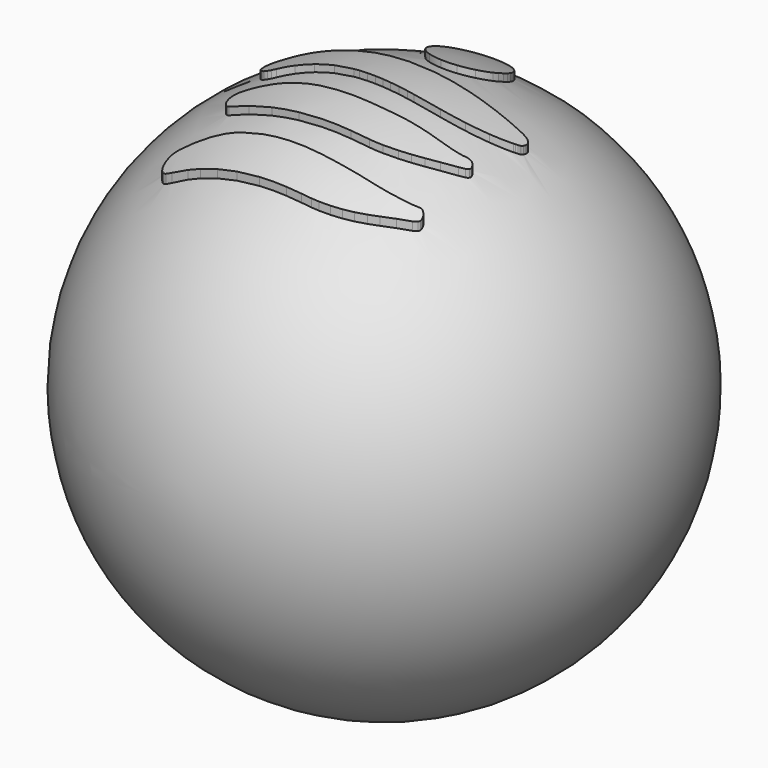
from build123d import *

# Parameters (mm, degrees)
F2_SCALE  = 33.3
F4_DEPTH  = 350
F5_SCALE  = 0.03
F8_SCALE  = 1.4
F9_R      = 2
F10_DEPTH = 25


# Not quite as in the source:
# - ends of sketch curves that miss each other by under 0.0002 mm in the source are joined


with BuildPart() as f1:
    # F0 (on Top) → F1 (revolve)
    with BuildSketch(Plane.XY):
        with BuildLine():
            ThreePointArc((0, 10), (-10, 0), (0, -10))
            Line((0, -10), (0, 10))
        make_face()
    revolve(axis=Axis((0, 0, 0), (0, 1, 0)))


with BuildPart() as f1_1:
    # F2: moved
    add(f1.part.scale(F2_SCALE))

    # F3 (on Top) → F4 (join)
    with BuildSketch(Plane.XY):
        with BuildLine():
            ThreePointArc((12.2771709421, 171.2973365957), (3.7569620218, 171.6476586922), (-4.6595689443, 170.277004793))
            ThreePointArc((-4.6595689443, 170.277004793), (-7.5791100861, 169.3858337465), (-10.4323080104, 168.3008600248))
            ThreePointArc((-10.4323080104, 168.3008600248), (-13.1062595865, 167.0608763501), (-15.6804411014, 165.6252001669))
            ThreePointArc((-15.6804411014, 165.6252001669), (-18.1927436184, 163.9705598843), (-20.5780995786, 162.1376454911))
            ThreePointArc((-20.5780995786, 162.1376454911), (-23.0057078919, 160.0044919193), (-25.3039240862, 157.7325260822))
            ThreePointArc((-25.3039240862, 157.7325260822), (-31.4706435539, 149.5429428278), (-35.5823828621, 140.1519202632))
            ThreePointArc((-35.5823828621, 140.1519202632), (-37.4151892223, 130.0698191221), (-36.8703758239, 119.8369740302))
            ThreePointArc((-36.8703758239, 119.8369740302), (-33.9846977784, 110.064148575), (-28.9042597875, 101.231006158))
            ThreePointArc((-28.9042597875, 101.231006158), (-21.9341856583, 93.8809503165), (-13.4222481029, 88.3898507888))
            ThreePointArc((-13.4222481029, 88.3898507888), (-4.5185212712, 85.102515885), (4.8600680158, 83.6447832896))
            ThreePointArc((4.8600680158, 83.6447832896), (14.0939838139, 84.1373624142), (23.0089839769, 86.5930920584))
            ThreePointArc((23.0089839769, 86.5930920584), (31.1392203878, 90.8795330247), (38.1542056195, 96.8179083614))
            ThreePointArc((38.1542056195, 96.8179083614), (43.8705462201, 104.2320953563), (47.9516467312, 112.6577310976))
            ThreePointArc((47.9516467312, 112.6577310976), (48.8982272616, 115.6703959892), (49.5778582503, 118.7542679562))
            ThreePointArc((49.5778582503, 118.7542679562), (50.0798461554, 122.2623063465), (50.3633334308, 125.7947219788))
            ThreePointArc((50.3633334308, 125.7947219788), (50.4261018055, 129.3073679001), (50.2697793114, 132.8170950236))
            ThreePointArc((50.2697793114, 132.8170950236), (49.8951754848, 135.8589541026), (49.2377071499, 138.8524420404))
            ThreePointArc((49.2377071499, 138.8524420404), (46.1875865729, 146.903977746), (41.6119908777, 154.1974259052))
            ThreePointArc((41.6119908777, 154.1974259052), (35.6444598617, 160.535838967), (28.5782016668, 165.6206104285))
            ThreePointArc((28.5782016668, 165.6206104285), (20.7020851759, 169.246924922), (12.2771709421, 171.2973365957))
        make_face()
        with BuildLine():
            ThreePointArc((-33.4008129923, 51.5219321661), (-43.3379692113, 51.2871840578), (-53.2641999456, 50.7655291885))
            ThreePointArc((-53.2641999456, 50.7655291885), (-64.0634546333, 49.7946073584), (-74.8074670149, 48.3342000935))
            ThreePointArc((-74.8074670149, 48.3342000935), (-84.6019065539, 46.4806697779), (-94.2713978098, 44.0583653252))
            ThreePointArc((-94.2713978098, 44.0583653252), (-102.9502181591, 41.3096782732), (-111.4351770957, 38.0107882245))
            ThreePointArc((-111.4351770957, 38.0107882245), (-118.9134806404, 34.4416572483), (-126.0622642904, 30.2513574505))
            ThreePointArc((-126.0622642904, 30.2513574505), (-129.4839108419, 27.8830120895), (-132.7427949411, 25.2952719306))
            ThreePointArc((-132.7427949411, 25.2952719306), (-136.5624533286, 21.9314871763), (-140.2579578012, 18.4317607976))
            ThreePointArc((-140.2579578012, 18.4317607976), (-143.6296449821, 15.0083482177), (-146.8849228402, 11.4740598577))
            ThreePointArc((-146.8849228402, 11.4740598577), (-148.6323854344, 9.2041815586), (-150.0384499195, 6.708393962))
            ThreePointArc((-150.0384499195, 6.708393962), (-151.1248140292, 3.7850161288), (-151.6963890826, 0.7191350082))
            ThreePointArc((-151.6963890826, 0.7191350082), (-151.7030139521, -2.2793436124), (-151.1351933539, -5.2235748094))
            ThreePointArc((-151.1351933539, -5.2235748094), (-150.0467353665, -7.8799584996), (-148.4426870406, -10.2607450339))
            ThreePointArc((-148.4426870406, -10.2607450339), (-146.4179490275, -12.215036049), (-144.0207902095, -13.6889584416))
            ThreePointArc((-144.0207902095, -13.6889584416), (-142.0108708561, -14.4907449782), (-139.9155901202, -15.0315186278))
            ThreePointArc((-139.9155901202, -15.0315186278), (-137.7958970772, -15.293695428), (-135.6601379416, -15.2745057775))
            ThreePointArc((-135.6601379416, -15.2745057775), (-133.3645757175, -14.9639575717), (-131.1220680921, -14.3832637152))
            ThreePointArc((-131.1220680921, -14.3832637152), (-128.6064090717, -13.4609337915), (-126.1693221699, -12.3474526631))
            ThreePointArc((-126.1693221699, -12.3474526631), (-117.4563433673, -8.4118226468), (-108.438275266, -5.2369791266))
            ThreePointArc((-108.438275266, -5.2369791266), (-98.1841126833, -2.4617275134), (-87.7763850745, -0.3335645669))
            ThreePointArc((-87.7763850745, -0.3335645669), (-76.345030466, 1.2950565214), (-64.8387360221, 2.2612154025))
            ThreePointArc((-64.8387360221, 2.2612154025), (-52.5535288324, 2.6415600166), (-40.2641999843, 2.433295384))
            ThreePointArc((-40.2641999843, 2.433295384), (-36.3905832333, 2.2574401909), (-32.5186950296, 2.0469324971))
            ThreePointArc((-32.5186950296, 2.0469324971), (-27.3626976167, 1.7334768445), (-22.2079499558, 1.4000996639))
            ThreePointArc((-22.2079499558, 1.4000996639), (-16.7235702373, 1.0242285256), (-11.2406670531, 0.6274002856))
            ThreePointArc((-11.2406670531, 0.6274002856), (-6.2514307284, 0.2440051169), (-1.2641999653, -0.1646515892))
            ThreePointArc((-1.2641999653, -0.1646515892), (3.8101984491, -0.5833479876), (8.8862039893, -0.9820881394))
            ThreePointArc((8.8862039893, -0.9820881394), (14.639141156, -1.4147968145), (20.3932289958, -1.8319250593))
            ThreePointArc((20.3932289958, -1.8319250593), (25.9302711121, -2.2181900783), (31.4683470454, -2.5893383091))
            ThreePointArc((31.4683470454, -2.5893383091), (35.8161186925, -2.8625927177), (40.1653459756, -3.111607448))
            ThreePointArc((40.1653459756, -3.111607448), (56.9461627797, -3.5511784434), (73.7250590157, -3.0435602691))
            ThreePointArc((73.7250590157, -3.0435602691), (87.9842368242, -1.5615103417), (102.051928967, 1.1990441357))
            ThreePointArc((102.051928967, 1.1990441357), (114.1685337399, 4.8311708126), (125.8390411692, 9.7100756482))
            ThreePointArc((125.8390411692, 9.7100756482), (136.1926279762, 15.5230963814), (145.7300484377, 22.5959726658))
            ThreePointArc((145.7300484377, 22.5959726658), (146.550290507, 23.3101400968), (147.3486982293, 24.0486367595))
            ThreePointArc((147.3486982293, 24.0486367595), (148.1402478445, 24.8249059327), (148.9094560487, 25.6233189544))
            ThreePointArc((148.9094560487, 25.6233189544), (149.5709024329, 26.3502366545), (150.2112826843, 27.0957792634))
            ThreePointArc((150.2112826843, 27.0957792634), (150.6030770817, 27.6129066708), (150.9446144028, 28.1645187761))
            ThreePointArc((150.9446144028, 28.1645187761), (151.5239999447, 29.4421682368), (151.887939637, 30.7970200663))
            ThreePointArc((151.887939637, 30.7970200663), (152.1005515096, 32.4270102974), (152.1458885281, 34.0701829889))
            ThreePointArc((152.1458885281, 34.0701829889), (152.0249488316, 35.6774007081), (151.7389896858, 37.2635919264))
            ThreePointArc((151.7389896858, 37.2635919264), (151.3206994021, 38.5039844833), (150.6750962556, 39.642728179))
            ThreePointArc((150.6750962556, 39.642728179), (149.4466397487, 41.0713121268), (147.9606871699, 42.2297172692))
            ThreePointArc((147.9606871699, 42.2297172692), (146.1844598756, 43.1548672571), (144.2800719274, 43.7746996926))
            ThreePointArc((144.2800719274, 43.7746996926), (141.3104289541, 44.3482005482), (138.3037060219, 44.6757673241))
            ThreePointArc((138.3037060219, 44.6757673241), (132.5218972582, 45.0258497218), (126.7358000073, 45.2959401848))
            ThreePointArc((126.7358000073, 45.2959401848), (122.2434994951, 45.4817627119), (117.7518210141, 45.6820583056))
            ThreePointArc((117.7518210141, 45.6820583056), (110.7327238683, 46.0095574172), (103.7139249982, 46.3433879632))
            ThreePointArc((103.7139249982, 46.3433879632), (95.7766243193, 46.7281179043), (87.8396770147, 47.1200702955))
            ThreePointArc((87.8396770147, 47.1200702955), (80.0375486713, 47.5126727242), (72.2358000183, 47.9127493529))
            ThreePointArc((72.2358000183, 47.9127493529), (47.9771765909, 49.1252386442), (23.714403985, 50.2516516642))
            ThreePointArc((23.714403985, 50.2516516642), (7.3055536967, 50.8943151333), (-9.1093480016, 51.3573339307))
            ThreePointArc((-9.1093480016, 51.3573339307), (-21.2544240802, 51.5365077254), (-33.4008129923, 51.5219321661))
        make_face()
        with BuildLine():
            ThreePointArc((135.3719059726, -35.3477778582), (133.7818150804, -35.7341828726), (132.2357999771, -36.2704059429))
            ThreePointArc((132.2357999771, -36.2704059429), (128.8416633612, -37.4833877287), (125.3645320803, -38.4326223458))
            ThreePointArc((125.3645320803, -38.4326223458), (121.5804634451, -39.1872771875), (117.7566089761, -39.7038197692))
            ThreePointArc((117.7566089761, -39.7038197692), (112.4926277716, -40.144911978), (107.2155060146, -40.3816535735))
            ThreePointArc((107.2155060146, -40.3816535735), (98.4763113976, -40.5631318855), (89.7358000012, -40.6627181729))
            ThreePointArc((89.7358000012, -40.6627181729), (84.01711687, -40.7186101274), (78.2988839889, -40.8095684171))
            ThreePointArc((78.2988839889, -40.8095684171), (72.2794587222, -40.9395955211), (66.2608000019, -41.101258064))
            ThreePointArc((66.2608000019, -41.101258064), (60.7936656268, -41.2769639411), (55.3275380245, -41.4816096107))
            ThreePointArc((55.3275380245, -41.4816096107), (51.5300788633, -41.6626782072), (47.7357999863, -41.9012778052))
            ThreePointArc((47.7357999863, -41.9012778052), (43.1515752062, -42.1702788658), (38.5622899772, -42.3313360205))
            ThreePointArc((38.5622899772, -42.3313360205), (33.1237885443, -42.4194447684), (27.6845839986, -42.4301682736))
            ThreePointArc((27.6845839986, -42.4301682736), (20.7404690874, -42.3574846085), (13.7975220184, -42.2108533058))
            ThreePointArc((13.7975220184, -42.2108533058), (4.3627493299, -41.9408030491), (-5.0707599904, -41.6297327271))
            ThreePointArc((-5.0707599904, -41.6297327271), (-26.6475844392, -41.0868134963), (-48.230946998, -40.9746754186))
            ThreePointArc((-48.230946998, -40.9746754186), (-63.0735777451, -41.481602722), (-77.8608920869, -42.8585552925))
            ThreePointArc((-77.8608920869, -42.8585552925), (-89.8112490712, -44.8116740031), (-101.5684681931, -47.7088283319))
            ThreePointArc((-101.5684681931, -47.7088283319), (-113.3171228374, -51.5855342168), (-124.7439711368, -56.3275667023))
            ThreePointArc((-124.7439711368, -56.3275667023), (-127.9028268029, -57.8339927228), (-131.0172902293, -59.430177568))
            ThreePointArc((-131.0172902293, -59.430177568), (-132.9810918572, -60.5975202718), (-134.8228720469, -61.9492049421))
            ThreePointArc((-134.8228720469, -61.9492049421), (-136.1124133389, -63.1590234551), (-137.2150186943, -64.5413545237))
            ThreePointArc((-137.2150186943, -64.5413545237), (-138.1156683785, -66.0761355261), (-138.791250415, -67.722437863))
            ThreePointArc((-138.791250415, -67.722437863), (-139.2810782207, -70.2023247824), (-139.1483839976, -72.7266389996))
            ThreePointArc((-139.1483839976, -72.7266389996), (-138.403814636, -75.611114725), (-137.2292449029, -78.3488089493))
            ThreePointArc((-137.2292449029, -78.3488089493), (-135.619610372, -80.9374429945), (-133.6426756543, -83.2577186477))
            ThreePointArc((-133.6426756543, -83.2577186477), (-131.5483835845, -84.9640158721), (-129.1400349314, -86.1876848195))
            ThreePointArc((-129.1400349314, -86.1876848195), (-128.2629859699, -86.4357293569), (-127.356108997, -86.5269167627))
            ThreePointArc((-127.356108997, -86.5269167627), (-114.4317156673, -86.6858032022), (-101.5072539913, -86.8390292524))
            ThreePointArc((-101.5072539913, -86.8390292524), (-86.9222267654, -86.988504971), (-72.3368410018, -87.0975202885))
            ThreePointArc((-72.3368410018, -87.0975202885), (-55.2271894087, -87.1869191844), (-38.117409, -87.2467869998))
            ThreePointArc((-38.117409, -87.2467869998), (-5.0620015712, -87.3020752377), (27.9934509997, -87.2935667483))
            ThreePointArc((27.9934509997, -87.2935667483), (39.5355017159, -87.1130359095), (51.0675479802, -86.5997766638))
            ThreePointArc((51.0675479802, -86.5997766638), (58.5947375628, -85.8686918997), (66.0448829765, -84.5693068899))
            ThreePointArc((66.0448829765, -84.5693068899), (74.2567660019, -82.5785408227), (82.348080106, -80.1436263203))
            ThreePointArc((82.348080106, -80.1436263203), (88.5910268151, -77.9251866229), (94.7309119323, -75.4356748429))
            ThreePointArc((94.7309119323, -75.4356748429), (101.0559287104, -72.5647344566), (107.2673301269, -69.455614242))
            ThreePointArc((107.2673301269, -69.455614242), (114.0377039152, -65.7576203133), (120.6797333565, -61.833774581))
            ThreePointArc((120.6797333565, -61.833774581), (128.26269397, -57.0666503711), (135.7409971679, -52.1369702488))
            ThreePointArc((135.7409971679, -52.1369702488), (138.6509308289, -50.0661186156), (141.4542029274, -47.8530199126))
            ThreePointArc((141.4542029274, -47.8530199126), (142.8833968287, -46.3593380839), (143.936998736, -44.580685882))
            ThreePointArc((143.936998736, -44.580685882), (144.3149857179, -43.0164260913), (144.106798527, -41.4206688294))
            ThreePointArc((144.106798527, -41.4206688294), (143.2964501997, -39.5119270792), (142.1632203142, -37.7753357528))
            ThreePointArc((142.1632203142, -37.7753357528), (141.304416429, -36.8626957087), (140.2983385608, -36.1155257159))
            ThreePointArc((140.2983385608, -36.1155257159), (139.215438827, -35.5919882204), (138.0501379645, -35.293932234))
            ThreePointArc((138.0501379645, -35.293932234), (136.7087205852, -35.2063854564), (135.3719059726, -35.3477778582))
        make_face()
        with BuildLine():
            ThreePointArc((138.362938908, -115.5407467287), (136.7862430463, -116.1135186456), (135.2357998792, -116.7539587246))
            ThreePointArc((135.2357998792, -116.7539587246), (132.4923488211, -117.8527968826), (129.6835140668, -118.771718229))
            ThreePointArc((129.6835140668, -118.771718229), (125.4590399229, -119.9562788795), (121.2108390004, -121.0527070018))
            ThreePointArc((121.2108390004, -121.0527070018), (116.5527038882, -122.1514879472), (111.8724679495, -123.1519547509))
            ThreePointArc((111.8724679495, -123.1519547509), (107.5493710974, -123.967786067), (103.2057619966, -124.666217977))
            ThreePointArc((103.2057619966, -124.666217977), (96.1817699296, -125.5240786292), (89.1243410013, -126.0389440267))
            ThreePointArc((89.1243410013, -126.0389440267), (78.3486567023, -126.4829388792), (67.5676439988, -126.7697639369))
            ThreePointArc((67.5676439988, -126.7697639369), (55.7624219473, -126.9096840156), (43.9564260012, -126.8735588899))
            ThreePointArc((43.9564260012, -126.8735588899), (33.0930358199, -126.6554595348), (22.2357999854, -126.2297323))
            ThreePointArc((22.2357999854, -126.2297323), (0.6169360978, -125.2847081037), (-21.0103899989, -124.5586829601))
            ThreePointArc((-21.0103899989, -124.5586829601), (-37.488469685, -124.2746975874), (-53.9687660125, -124.3618242436))
            ThreePointArc((-53.9687660125, -124.3618242436), (-66.7788526349, -124.7610039981), (-79.5718179796, -125.5341152714))
            ThreePointArc((-79.5718179796, -125.5341152714), (-89.4597028969, -126.5838489133), (-99.2642000856, -128.2403645735))
            ThreePointArc((-99.2642000856, -128.2403645735), (-106.5112517599, -129.8844871019), (-113.6674199964, -131.8875230116))
            ThreePointArc((-113.6674199964, -131.8875230116), (-121.7495540082, -134.5168586664), (-129.7394031383, -137.4145486376))
            ThreePointArc((-129.7394031383, -137.4145486376), (-137.0035815143, -140.2947890599), (-144.191216808, -143.3610524345))
            ThreePointArc((-144.191216808, -143.3610524345), (-147.1391871622, -145.0946267516), (-149.6119794457, -147.45706346))
            ThreePointArc((-149.6119794457, -147.45706346), (-150.8691223595, -149.3653302628), (-151.6786876083, -151.5022661008))
            ThreePointArc((-151.6786876083, -151.5022661008), (-152.0975766592, -153.9721486933), (-152.0978704949, -156.4773010416))
            ThreePointArc((-152.0978704949, -156.4773010416), (-151.6677822056, -159.1101873912), (-150.83334997, -161.6441149874))
            ThreePointArc((-150.83334997, -161.6441149874), (-149.6081984193, -164.0438572615), (-148.034591302, -166.2309832541))
            ThreePointArc((-148.034591302, -166.2309832541), (-146.1550700782, -168.1201321526), (-143.9881808848, -169.6712848069))
            ThreePointArc((-143.9881808848, -169.6712848069), (-141.7301714831, -170.7237495772), (-139.3060209204, -171.2980163953))
            ThreePointArc((-139.3060209204, -171.2980163953), (-135.3926491876, -171.6566898855), (-131.463183991, -171.7059703329))
            ThreePointArc((-131.463183991, -171.7059703329), (-121.501850768, -171.4036347719), (-111.5428429878, -171.0325143005))
            ThreePointArc((-111.5428429878, -171.0325143005), (-103.7628838008, -170.7645404312), (-95.9801760095, -170.594145395))
            ThreePointArc((-95.9801760095, -170.594145395), (-85.5050870543, -170.4580843566), (-75.0294270049, -170.3771660432))
            ThreePointArc((-75.0294270049, -170.3771660432), (-62.4856587788, -170.3422457704), (-49.9418629992, -170.3652268177))
            ThreePointArc((-49.9418629992, -170.3652268177), (-35.6028707395, -170.4467996665), (-21.2642000002, -170.572794018))
            ThreePointArc((-21.2642000002, -170.572794018), (-3.9936634451, -170.7363721352), (13.2771299946, -170.8701057803))
            ThreePointArc((13.2771299946, -170.8701057803), (22.738108269, -170.8919091414), (32.1988900013, -170.8271461173))
            ThreePointArc((32.1988900013, -170.8271461173), (38.2944995089, -170.7075579335), (44.3873299873, -170.4880737132))
            ThreePointArc((44.3873299873, -170.4880737132), (48.7220290947, -170.2010087405), (53.0399790565, -169.7242164257))
            ThreePointArc((53.0399790565, -169.7242164257), (59.6595394202, -168.716160739), (66.2354630286, -167.4544221349))
            ThreePointArc((66.2354630286, -167.4544221349), (72.4172358028, -165.998419384), (78.5271688779, -164.2655096038))
            ThreePointArc((78.5271688779, -164.2655096038), (84.5465659654, -162.2611361163), (90.4694701318, -159.9874033215))
            ThreePointArc((90.4694701318, -159.9874033215), (96.5964383825, -157.3357343833), (102.6161871077, -154.4489172139))
            ThreePointArc((102.6161871077, -154.4489172139), (108.0505025631, -151.5873003946), (113.3772680483, -148.5301440807))
            ThreePointArc((113.3772680483, -148.5301440807), (120.3987931958, -144.2547366455), (127.3532623778, -139.8710985893))
            ThreePointArc((127.3532623778, -139.8710985893), (134.1241029841, -135.4830989804), (140.8520629258, -131.029630889))
            ThreePointArc((140.8520629258, -131.029630889), (143.0569157896, -129.3075952587), (144.9857997246, -127.2812217739))
            ThreePointArc((144.9857997246, -127.2812217739), (145.6313821073, -126.2754391513), (146.0270038801, -125.1476719731))
            ThreePointArc((146.0270038801, -125.1476719731), (146.2047673588, -123.8353991816), (146.154986262, -122.5120769674))
            ThreePointArc((146.154986262, -122.5120769674), (145.8707377397, -121.1425533571), (145.3695139558, -119.8367330212))
            ThreePointArc((145.3695139558, -119.8367330212), (144.6703164334, -118.6486179488), (143.7812548902, -117.5950221098))
            ThreePointArc((143.7812548902, -117.5950221098), (142.8320627321, -116.7196961588), (141.8152178843, -115.9239651608))
            ThreePointArc((141.8152178843, -115.9239651608), (141.0626237676, -115.5204237855), (140.2310500198, -115.3261847988))
            ThreePointArc((140.2310500198, -115.3261847988), (139.285554859, -115.333865295), (138.362938908, -115.5407467287))
        make_face()
    extrude(amount=F4_DEPTH)


with BuildPart() as f1_2:
    # F5: moved
    add(f1_1.part.scale(F5_SCALE))

    # F6 (on Top) → F7 (revolve, cut)
    with BuildSketch(Plane.XY):
        with BuildLine():
            Line((0, 10.25), (0, 15))
            ThreePointArc((0, 15), (-15, 0), (0, -15))
            Line((0, -15), (0, -10.25))
            ThreePointArc((0, -10.25), (-10.25, 0), (0, 10.25))
        make_face()
        with BuildLine():
            Line((0, -7), (0, 7))
            ThreePointArc((0, 7), (-7, 0), (0, -7))
        make_face()
    revolve(axis=Axis((0, 0, 0), (0, -1, 0)), mode=Mode.SUBTRACT)


with BuildPart() as f1_3:
    # F8: moved
    add(f1_2.part.scale(F8_SCALE))

    # F9 (on Front) → F10 (cut)
    with BuildSketch(Plane.XZ):
        with Locations((0, -5.1200183504)):
            Circle(F9_R)
    extrude(amount=-F10_DEPTH, mode=Mode.SUBTRACT)


solid = f1_3.part
